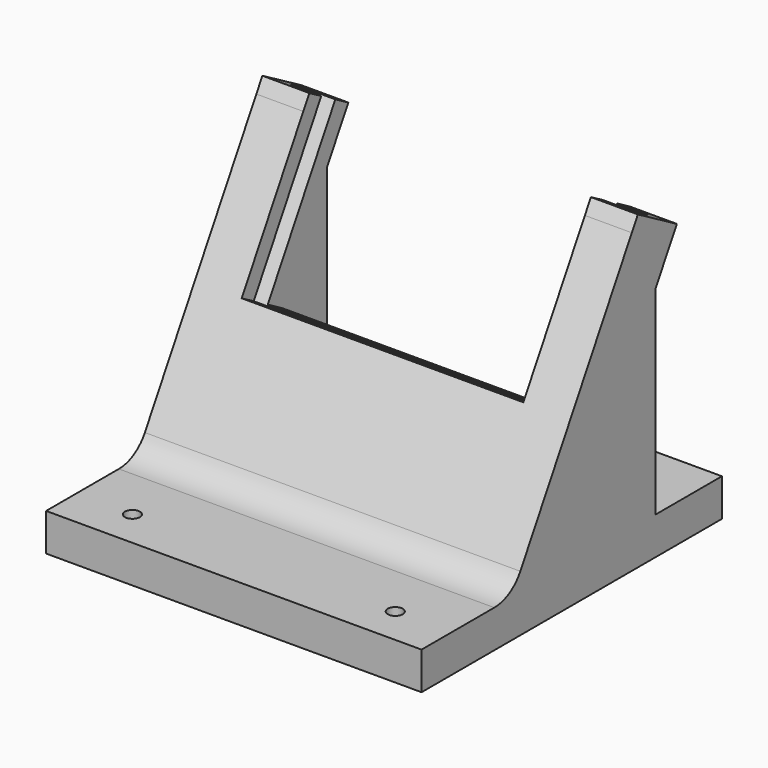
from build123d import *

# Parameters (mm, degrees)
F1_DEPTH      = 127
F2_W          = 95.25
F2_H          = 57.15
F3_DEPTH      = 83.3406583964
F4_R          = 2.54
F5_DEPTH      = 12.701
F6_R          = 2.54
F7_DEPTH      = 12.701
F8_W          = 106.045
F8_H          = 6.858
F8_W_2        = 10.795
F9_DEPTH      = 59.69
F10_W         = 95.25
F10_H         = 22.0760425496
F10_H_2       = 18.8356010627
F11_DEPTH     = 19.05
F12_W         = 119.38
F12_H         = 119.38
F12_R         = 6.35
F13_DEPTH     = 7.62
F14_T         = 5.08
F14_T3_DEPTH  = 17.78
F14_T5_DEPTH  = 26.035
F14_T7_DEPTH  = 29.21
F14_T9_DEPTH  = 105.41
F14_T11_DEPTH = 26.035
F14_T13_DEPTH = 17.1416638094
F14_T15_DEPTH = 43.2345651777
F14_T17_DEPTH = 16.002
F14_T19_DEPTH = 69.85
F14_T21_DEPTH = 127
F14_T23_DEPTH = 17.018
F14_T25_DEPTH = 17.018


# Not quite as in the source:
# - a shell that OpenCascade refuses in one call is made with other operations: the cavity is built on its own and cut out


with BuildPart() as f1:
    # F0 (on Right) → F1 (new body)
    with BuildSketch(Plane.YZ):
        with BuildLine():
            Line((0, 12.7), (0, 0))
            Line((0, 0), (127, 0))
            Line((127, 0), (127, 12.7))
            Line((127, 12.7), (98.9720369056, 12.7))
            Line((98.9720369056, 12.7), (98.9720369056, 80.0334606807))
            Line((98.9720369056, 80.0334606807), (107.95, 95.5837489087))
            Line((107.95, 95.5837489087), (91.4522160579, 105.1087489087))
            Line((91.4522160579, 105.1087489087), (88.9, 100.6881810245))
            Line((88.9, 100.6881810245), (41.7661742094, 19.05))
            ThreePointArc((41.7661742094, 19.05), (37.1176515813, 14.4014773719), (30.7676515813, 12.7))
            Line((30.7676515813, 12.7), (0, 12.7))
        make_face()
    extrude(amount=F1_DEPTH)

    # F2 (on face) → F3 (cut, through all)
    with BuildSketch(Plane(origin=(0, 23.075738686, -13.3227839421), x_dir=(1, 0, 0), z_dir=(0, -0.8660254038, 0.5))):
        with Locations((63.5, 108.1779547439)):
            Rectangle(F2_W, F2_H)
    extrude(amount=-F3_DEPTH, mode=Mode.SUBTRACT)

    # F4 (on face) → F5 (cut, through all)
    with BuildSketch(Plane.XY.offset(12.7)):
        with Locations((19.05, 12.7)):
            Circle(F4_R)
        with Locations((107.95, 12.7)):
            Circle(F4_R)
    extrude(amount=-F5_DEPTH, mode=Mode.SUBTRACT)

    # F6 (on face) → F7 (cut, through all)
    with BuildSketch(Plane.XY.offset(12.7)):
        with Locations((19.05, 114.3)):
            Circle(F6_R)
        with Locations((107.95, 114.3)):
            Circle(F6_R)
    extrude(amount=-F7_DEPTH, mode=Mode.SUBTRACT)

    # F8 (on face) → F9 (cut)
    with BuildSketch(Plane(origin=(0, 68.3764773719, 118.4315328508), x_dir=(1, 0, 0), z_dir=(0, 0.5, 0.8660254038))):
        with Locations((58.1025, 35.9165678842)):
            Rectangle(F8_W, F8_H)
        with Locations((116.5225, 35.9165678842)):
            Rectangle(F8_W_2, F8_H)
    extrude(amount=-F9_DEPTH, mode=Mode.SUBTRACT)

    # F10 (on face) → F11 (cut)
    with BuildSketch(Plane(origin=(0, 98.9720369056, 0), x_dir=(-1, 0, 0), z_dir=(0, 1, 0))):
        with Locations((-63.5, 23.7380212748)):
            Rectangle(F10_W, F10_H)
        with Locations((-63.5, 44.193843081)):
            Rectangle(F10_W, F10_H_2)
    extrude(amount=-F11_DEPTH, mode=Mode.SUBTRACT)

    # F12 (on face) → F13 (cut)
    with BuildSketch(Plane(origin=(0, 0, 0), x_dir=(1, 0, 0), z_dir=(0, 0, -1))):
        with Locations((63.5, -63.5)):
            Rectangle(F12_W, F12_H)
        with Locations((19.05, -114.3)):
            Circle(F12_R, mode=Mode.SUBTRACT)
        with Locations((107.95, -114.3)):
            Circle(F12_R, mode=Mode.SUBTRACT)
        with Locations((19.05, -12.7)):
            Circle(F12_R, mode=Mode.SUBTRACT)
        with Locations((107.95, -12.7)):
            Circle(F12_R, mode=Mode.SUBTRACT)
    extrude(amount=-F13_DEPTH, mode=Mode.SUBTRACT)

    # F14: shell of thickness 5.08, made by hand


with BuildPart() as f14_core1:
    # F14_t2: copy of F1
    add(f1.part)

    # the walls: a layer under each face that stays
    f14_faces = [f14_core1.faces().sort_by_distance(p)[0] for p in [
        (63.5, 0, 6.35),
        (63.5, 15.3838257906, 12.7),
        (125.4320987654, 107.15625, 0),
        (0, 63.5, 52.5543744543),
        (127, 63.5, 52.5543744543),
        (63.5, 37.1176515813, 14.4014773719),
        (105.41, 12.7, 6.35),
        (16.51, 12.7, 6.35),
        (63.5, 127, 6.35),
        (3.81, 63.5, 3.81),
        (63.5, 3.81, 3.81),
        (123.19, 63.5, 3.81),
        (63.5, 123.19, 3.81),
        (63.5, 103.4610184528, 12.7),
        (7.9375, 98.9720369056, 46.3667303403),
        (7.9375, 103.4610184528, 87.8086047947),
        (13.2291666667, 105.200369343, 97.1712489087),
        (105.8333333333, 50.0471811841, 33.3931248181),
        (119.0625, 98.9720369056, 46.3667303403),
        (119.0625, 103.4610184528, 87.8086047947),
        (124.3541666667, 105.200369343, 97.1712489087),
        (112.1833333333, 8.4666666667, 0),
        (23.2833333333, 8.4666666667, 0),
        (111.125, 90.912869343, 55.7293744543),
        (63.5, 79.9220369056, 29.2372825889),
        (15.875, 98.3301377958, 51.6049284688),
        (105.41, 114.3, 6.35),
        (16.51, 114.3, 6.35),
        (15.875, 79.6943762624, 78.9015729955),
        (13.4257142857, 68.7983221811, 54.1870537248),
        (5.08, 84.5586375764, 74.6267207327),
        (113.5742857143, 74.7375244003, 50.7580537248),
        (111.125, 79.6943762624, 78.9015729955),
        (63.5, 65.4068762624, 54.1548970824),
        (121.92, 84.5586375764, 74.6267207327),
        (101.6, 12.7, 3.81),
        (12.7, 12.7, 3.81),
        (12.7, 114.3, 3.81),
        (101.6, 114.3, 3.81),
        (63.5, 76.8988877958, 47.5199811301),
        (112.1833333333, 110.0666666667, 0),
        (23.2833333333, 110.0666666667, 0),
        (63.5, 69.6361375764, 48.7801925568),
    ]]
    thicken(f14_faces, amount=-F14_T, mode=Mode.SUBTRACT)

    # F14_s4 → F14_t3 (cut)
    with BuildSketch(Plane.XY.offset(-5.08)):
        Polygon((3.8608, 3.8608), (-1.27, 3.81), (-1.27, -1.27), (3.81, -1.27), align=None)
        Polygon((3.8608, 123.1392), (-1.27, 123.19), (-1.27, 128.27), (3.81, 128.27), align=None)
        Polygon((123.1392, 3.8608), (123.19, -1.27), (128.27, -1.27), (128.27, 3.81), align=None)
        Polygon((123.1392, 123.1392), (128.27, 123.19), (128.27, 128.27), (123.19, 128.27), align=None)
    extrude(amount=F14_T3_DEPTH, mode=Mode.SUBTRACT)

    # F14_s6 → F14_t5 (cut)
    with BuildSketch(Plane.YZ.offset(106.045)):
        Polygon((99.0228369056, 12.7508), (98.9720369056, 7.62), (93.8920369056, 7.62), (93.8920369056, 12.7), align=None)
        Polygon((99.0668309961, 80.0080606807), (93.8920369056, 80.0334606807), (93.8920369056, 81.3946425782), (94.5726278544, 82.5734606807), align=None)
    extrude(amount=F14_T5_DEPTH, mode=Mode.SUBTRACT)

    # F14_s8 → F14_t7 (cut)
    with BuildSketch(Plane.XZ.offset(-104.0520369056)):
        Polygon((111.0742, 12.7508), (111.125, 7.62), (116.205, 7.62), (116.205, 12.7), align=None)
        Polygon((15.9258, 12.7508), (15.875, 7.62), (10.795, 7.62), (10.795, 12.7), align=None)
    extrude(amount=F14_T7_DEPTH, mode=Mode.SUBTRACT)

    # F14_s10 → F14_t9 (cut)
    with BuildSketch(Plane.YZ.offset(10.795)):
        Polygon((79.9728369056, 12.7508), (79.9220369056, 7.62), (74.8420369056, 7.62), (74.8420369056, 12.7), align=None)
    extrude(amount=F14_T9_DEPTH, mode=Mode.SUBTRACT)

    # F14_s12 → F14_t11 (cut)
    with BuildSketch(Plane.YZ.offset(-5.08)):
        Polygon((99.0228369056, 12.7508), (98.9720369056, 7.62), (93.8920369056, 7.62), (93.8920369056, 12.7), align=None)
        Polygon((99.0668309961, 80.0080606807), (93.8920369056, 80.0334606807), (93.8920369056, 81.3946425782), (94.5726278544, 82.5734606807), align=None)
    extrude(amount=F14_T11_DEPTH, mode=Mode.SUBTRACT)

    # F14_s14 → F14_t13 (cut)
    with BuildSketch(Plane(origin=(0, 29.6748522628, -17.1327839421), x_dir=(1, 0, 0), z_dir=(0, 0.8660254038, -0.5))):
        Polygon((111.0742, -79.6537547439), (116.205, -79.6029547439), (116.205, -74.5229547439), (111.125, -74.5229547439), align=None)
        Polygon((15.9258, -79.6537547439), (10.795, -79.6029547439), (10.795, -74.5229547439), (15.875, -74.5229547439), align=None)
    extrude(amount=F14_T13_DEPTH, mode=Mode.SUBTRACT)

    # F14_s16 → F14_t15 (cut)
    with BuildSketch(Plane.XY.offset(7.62)):
        Polygon((111.0742, 79.9728369056), (116.205, 79.9220369056), (116.205, 74.8420369056), (111.125, 74.8420369056), align=None)
        Polygon((15.9258, 79.9728369056), (15.875, 74.8420369056), (10.795, 74.8420369056), (10.795, 79.9220369056), align=None)
    extrude(amount=F14_T15_DEPTH, mode=Mode.SUBTRACT)

    # F14_s18 → F14_t17 (cut)
    with BuildSketch(Plane(origin=(0, 18.6763296347, -10.7827839421), x_dir=(1, 0, 0), z_dir=(0, 0.8660254038, -0.5))):
        Polygon((15.9258, -79.6537547439), (10.795, -79.6029547439), (10.795, -74.5229547439), (15.875, -74.5229547439), align=None)
        Polygon((111.0742, -79.6537547439), (116.205, -79.6029547439), (116.205, -74.5229547439), (111.125, -74.5229547439), align=None)
    extrude(amount=F14_T17_DEPTH, mode=Mode.SUBTRACT)

    # F14_s20 → F14_t19 (cut)
    with BuildSketch(Plane(origin=(0, 70.9164773719, 122.830941902), x_dir=(1, 0, 0), z_dir=(0, -0.5, -0.8660254038))):
        Polygon((121.8692, -32.5383678842), (121.92, -27.4075678842), (127, -27.4075678842), (127, -32.4875678842), align=None)
        Polygon((5.1308, -32.5383678842), (5.08, -27.4075678842), (0, -27.4075678842), (0, -32.4875678842), align=None)
        Polygon((5.1308, -39.2947678842), (0, -39.3455678842), (0, -44.4255678842), (5.08, -44.4255678842), align=None)
        Polygon((121.8692, -39.2947678842), (121.92, -44.4255678842), (127, -44.4255678842), (127, -39.3455678842), align=None)
    extrude(amount=F14_T19_DEPTH, mode=Mode.SUBTRACT)

    # F14_s22 → F14_t21 (cut)
    with BuildSketch(Plane.YZ):
        Polygon((66.7359305573, 50.5132866473), (62.2671274156, 53.0346925568), (59.7271274156, 48.6352835056), (64.1265364668, 46.0952835056), align=None)
        Polygon((72.5871445955, 47.1350866473), (77.0051477372, 44.5256925568), (74.4651477372, 40.1262835056), (70.065738686, 42.6662835056), align=None)
    extrude(amount=F14_T21_DEPTH, mode=Mode.SUBTRACT)

    # F14_s24 → F14_t23 (cut)
    with BuildSketch(Plane(origin=(0, 38.4736703653, -22.2127839421), x_dir=(1, 0, 0), z_dir=(0, -0.8660254038, 0.5))):
        Polygon((5.1308, 77.1137547439), (0, 77.0629547439), (0, 71.9829547439), (5.08, 71.9829547439), align=None)
    extrude(amount=F14_T23_DEPTH, mode=Mode.SUBTRACT)

    # F14_s26 → F14_t25 (cut)
    with BuildSketch(Plane(origin=(0, 23.7356500437, -13.7037839421), x_dir=(1, 0, 0), z_dir=(0, 0.8660254038, -0.5))):
        Polygon((121.8692, -77.1137547439), (127, -77.0629547439), (127, -71.9829547439), (121.92, -71.9829547439), align=None)
    extrude(amount=F14_T25_DEPTH, mode=Mode.SUBTRACT)


with BuildPart() as f1_1:
    add(f1.part)

    # what is left inside the walls is the cavity
    f14_cavity = [f14_core1.part.solids().sort_by_distance(p)[0] for p in [
        (63.5, 72.850575, 7.6708),
    ]]
    add(f14_cavity, mode=Mode.SUBTRACT)


solid = f1_1.part
